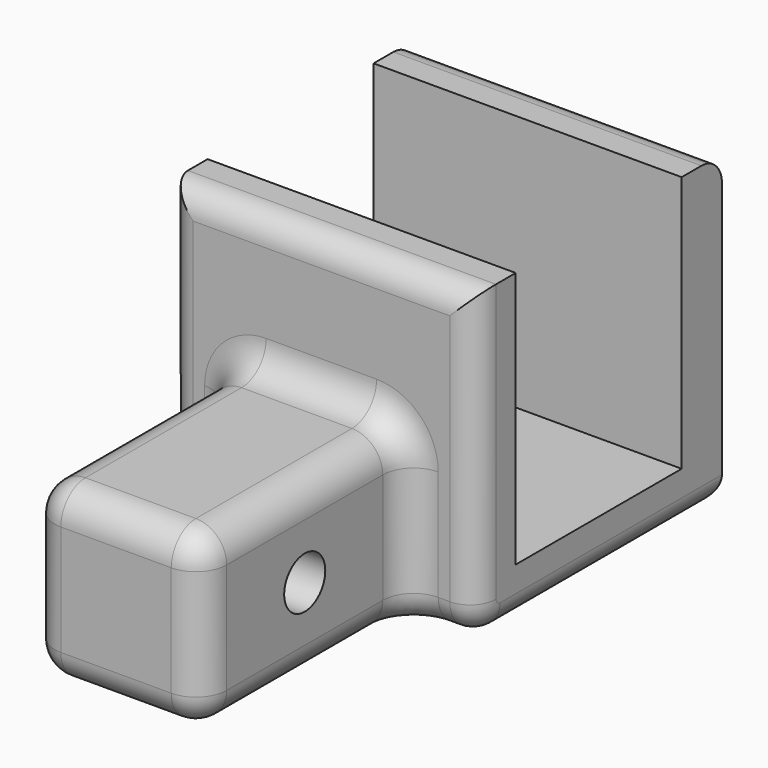
from build123d import *

# Parameters (mm, degrees)
F0_W      = 30
F0_H      = 30
F1_DEPTH  = 5
F2_W      = 30
F2_H      = 4.9
F3_DEPTH  = 25
F4_W      = 16.75
F4_H      = 16.75
F5_DEPTH  = 25
F6_R      = 3
F7_R      = 2.5
F9_R      = 2.5
F10_DEPTH = 16.75


# Not quite as in the source:
# - two fillets or chamfers of one size are made in one step
# - a feature names something its author has since deleted; it is built from what else it names


with BuildPart() as f1:
    # F0 (on Top) → F1 (new body)
    with BuildSketch(Plane.XY):
        with Locations((15, 15)):
            Rectangle(F0_W, F0_H)
    extrude(amount=F1_DEPTH)

    # F2 (on face) → F3 (join)
    with BuildSketch(Plane.XY.offset(5)):
        with Locations((15, 27.55)):
            Rectangle(F2_W, F2_H)
        with Locations((15, 2.45)):
            Rectangle(F2_W, F2_H)
    extrude(amount=F3_DEPTH)

    # F4 (on face) → F5 (join)
    with BuildSketch(Plane.XZ):
        with Locations((15, 8.375)):
            Rectangle(F4_W, F4_H)
    extrude(amount=F5_DEPTH)

    # F6
    f6_edges = [f1.edges().sort_by_distance(p)[0] for p in [
        (6.625, -25, 8.375),
        (23.375, 0, 8.375),
        (23.375, -12.5, 0),
        (23.375, -12.5, 16.75),
        (23.375, -25, 8.375),
        (3.3125, 0, 0),
        (6.625, 0, 8.375),
        (15, 0, 16.75),
        (26.6875, 0, 0),
        (6.625, -12.5, 0),
        (15, -25, 0),
        (6.625, -12.5, 16.75),
        (15, -25, 16.75),
    ]]
    fillet(f6_edges, radius=F6_R)

    # F7
    f7_edges = [f1.edges().sort_by_distance(p)[0] for p in [
        (15, 30, 30),
        (15, 0, 30),
        (15, 30, 0),
        (30, 16.5, 0),
        (0, 16.5, 0),
        (0, 0, 16.5),
        (0, 0.87868, 0.87868),
        (30, 0, 16.5),
        (30, 0.87868, 0.87868),
    ]]
    fillet(f7_edges, radius=F7_R)

    # F9 (on face) → F10 (cut, through all)
    with BuildSketch(Plane.YZ.offset(23.375)):
        with Locations((-12.5, 8.375)):
            Circle(F9_R)
    extrude(amount=-F10_DEPTH, mode=Mode.SUBTRACT)


solid = f1.part
